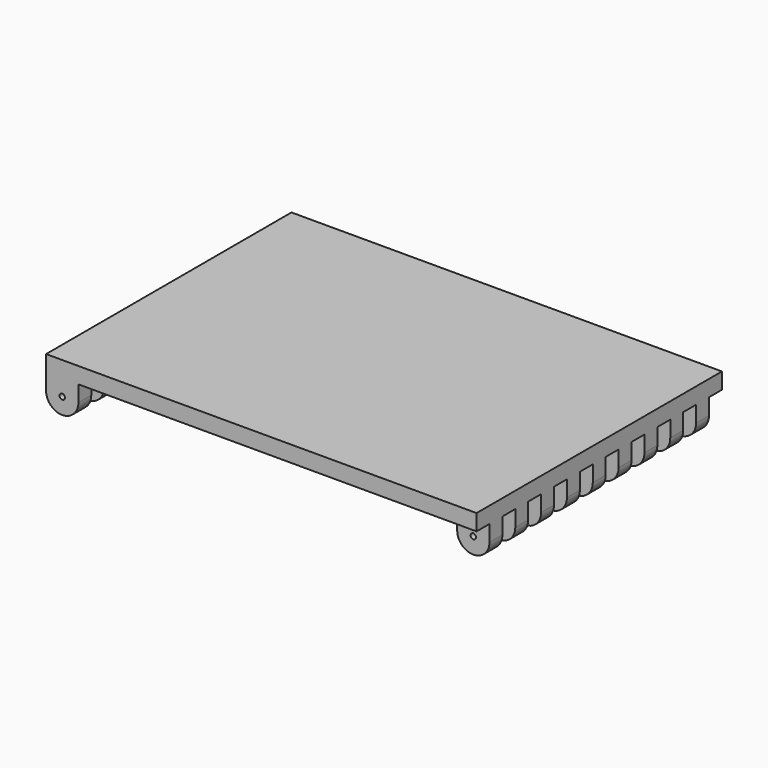
from build123d import *

# Parameters (mm, degrees)
F0_W      = 508
F0_H      = 361.95
F1_DEPTH  = 19.05
F2_W      = 38.1
F2_H      = 19.05
F3_DEPTH  = 38.1
F4_R      = 19.04999
F5_R      = 19.04999
F6_R      = 3.175
F7_DEPTH  = 361.951
F8_W      = 38.1
F8_H      = 38.1
F9_DEPTH  = 361.951
F10_W     = 38.1
F10_H     = 19.05
F11_DEPTH = 38.1
F12_R     = 19.04999
F13_R     = 3.175
F14_DEPTH = 342.901


# Not quite as in the source:
# - a fillet or chamfer is up to 0.001 mm smaller than in the source, because OpenCascade refuses the exact size


with BuildPart() as f1:
    # F0 (on Top) → F1 (new body)
    with BuildSketch(Plane.XY):
        with Locations((254, 180.975)):
            Rectangle(F0_W, F0_H)
    extrude(amount=F1_DEPTH)

    # F2 (on face) → F3 (join)
    with BuildSketch(Plane(origin=(0, 0, 0), x_dir=(1, 0, 0), z_dir=(0, 0, -1))):
        with Locations((19.05, -9.525)):
            Rectangle(F2_W, F2_H)
        with Locations((19.05, -47.625)):
            Rectangle(F2_W, F2_H)
        with Locations((19.05, -85.725)):
            Rectangle(F2_W, F2_H)
        with Locations((19.05, -123.825)):
            Rectangle(F2_W, F2_H)
        with Locations((19.05, -161.925)):
            Rectangle(F2_W, F2_H)
        with Locations((19.05, -200.025)):
            Rectangle(F2_W, F2_H)
        with Locations((19.05, -238.125)):
            Rectangle(F2_W, F2_H)
        with Locations((19.05, -276.225)):
            Rectangle(F2_W, F2_H)
        with Locations((19.05, -314.325)):
            Rectangle(F2_W, F2_H)
        with Locations((19.05, -352.425)):
            Rectangle(F2_W, F2_H)
        with Locations((488.95, -9.525)):
            Rectangle(F2_W, F2_H)
        with Locations((488.95, -47.625)):
            Rectangle(F2_W, F2_H)
        with Locations((488.95, -85.725)):
            Rectangle(F2_W, F2_H)
        with Locations((488.95, -123.825)):
            Rectangle(F2_W, F2_H)
        with Locations((488.95, -161.925)):
            Rectangle(F2_W, F2_H)
        with Locations((488.95, -200.025)):
            Rectangle(F2_W, F2_H)
        with Locations((488.95, -238.125)):
            Rectangle(F2_W, F2_H)
        with Locations((488.95, -276.225)):
            Rectangle(F2_W, F2_H)
        with Locations((488.95, -314.325)):
            Rectangle(F2_W, F2_H)
        with Locations((488.95, -352.425)):
            Rectangle(F2_W, F2_H)
    extrude(amount=F3_DEPTH)

    # F4 (radius 19.05 in the source; OpenCascade refuses exactly that, so slightly less here)
    f4_edges = [f1.edges().sort_by_distance(p)[0] for p in [
        (508, 9.525, -38.1),
        (469.9, 9.525, -38.1),
        (469.9, 47.625, -38.1),
        (508, 47.625, -38.1),
        (508, 85.725, -38.1),
        (469.9, 85.725, -38.1),
        (469.9, 123.825, -38.1),
        (508, 123.825, -38.1),
        (508, 161.925, -38.1),
        (469.9, 161.925, -38.1),
        (508, 200.025, -38.1),
        (469.9, 200.025, -38.1),
        (469.9, 238.125, -38.1),
        (508, 238.125, -38.1),
        (469.9, 276.225, -38.1),
        (508, 276.225, -38.1),
        (469.9, 314.325, -38.1),
        (508, 314.325, -38.1),
        (469.9, 352.425, -38.1),
        (508, 352.425, -38.1),
    ]]
    fillet(f4_edges, radius=F4_R)

    # F5 (radius 19.05 in the source; OpenCascade refuses exactly that, so slightly less here)
    f5_edges = [f1.edges().sort_by_distance(p)[0] for p in [
        (38.1, 9.525, -38.1),
        (0, 9.525, -38.1),
        (38.1, 47.625, -38.1),
        (0, 47.625, -38.1),
        (38.1, 85.725, -38.1),
        (0, 85.725, -38.1),
        (38.1, 123.825, -38.1),
        (0, 123.825, -38.1),
        (0, 161.925, -38.1),
        (38.1, 161.925, -38.1),
        (38.1, 200.025, -38.1),
        (0, 200.025, -38.1),
        (0, 238.125, -38.1),
        (38.1, 238.125, -38.1),
        (38.1, 276.225, -38.1),
        (0, 276.225, -38.1),
        (38.1, 314.325, -38.1),
        (0, 314.325, -38.1),
        (38.1, 352.425, -38.1),
        (0, 352.425, -38.1),
    ]]
    fillet(f5_edges, radius=F5_R)

    # F6 (on face) → F7 (cut, through all)
    with BuildSketch(Plane.XZ):
        with Locations((19.05, -19.05)):
            Circle(F6_R)
        with Locations((488.95, -19.05)):
            Circle(F6_R)
    extrude(amount=-F7_DEPTH, mode=Mode.SUBTRACT)

    # F8 (on face) → F9 (cut, through all)
    with BuildSketch(Plane.XZ):
        with Locations((488.95, -19.05)):
            Rectangle(F8_W, F8_H)
    extrude(amount=-F9_DEPTH, mode=Mode.SUBTRACT)

    # F10 (on face) → F11 (join)
    with BuildSketch(Plane(origin=(0, 0, 0), x_dir=(1, 0, 0), z_dir=(0, 0, -1))):
        with Locations((488.95, -28.575)):
            Rectangle(F10_W, F10_H)
        with Locations((488.95, -66.675)):
            Rectangle(F10_W, F10_H)
        with Locations((488.95, -104.775)):
            Rectangle(F10_W, F10_H)
        with Locations((488.95, -142.875)):
            Rectangle(F10_W, F10_H)
        with Locations((488.95, -180.975)):
            Rectangle(F10_W, F10_H)
        with Locations((488.95, -219.075)):
            Rectangle(F10_W, F10_H)
        with Locations((488.95, -257.175)):
            Rectangle(F10_W, F10_H)
        with Locations((488.95, -295.275)):
            Rectangle(F10_W, F10_H)
        with Locations((488.95, -333.375)):
            Rectangle(F10_W, F10_H)
    extrude(amount=F11_DEPTH)

    # F12 (radius 19.05 in the source; OpenCascade refuses exactly that, so slightly less here)
    f12_edges = [f1.edges().sort_by_distance(p)[0] for p in [
        (469.9, 28.575, -38.1),
        (508, 28.575, -38.1),
        (508, 66.675, -38.1),
        (508, 104.775, -38.1),
        (508, 142.875, -38.1),
        (508, 180.975, -38.1),
        (469.9, 66.675, -38.1),
        (469.9, 104.775, -38.1),
        (469.9, 142.875, -38.1),
        (469.9, 180.975, -38.1),
        (469.9, 219.075, -38.1),
        (469.9, 257.175, -38.1),
        (469.9, 295.275, -38.1),
        (469.9, 333.375, -38.1),
        (508, 333.375, -38.1),
        (508, 295.275, -38.1),
        (508, 219.075, -38.1),
        (508, 257.175, -38.1),
    ]]
    fillet(f12_edges, radius=F12_R)

    # F13 (on face) → F14 (cut, through all)
    with BuildSketch(Plane.XZ.offset(-19.05)):
        with Locations((488.95, -19.05)):
            Circle(F13_R)
    extrude(amount=-F14_DEPTH, mode=Mode.SUBTRACT)


solid = f1.part
